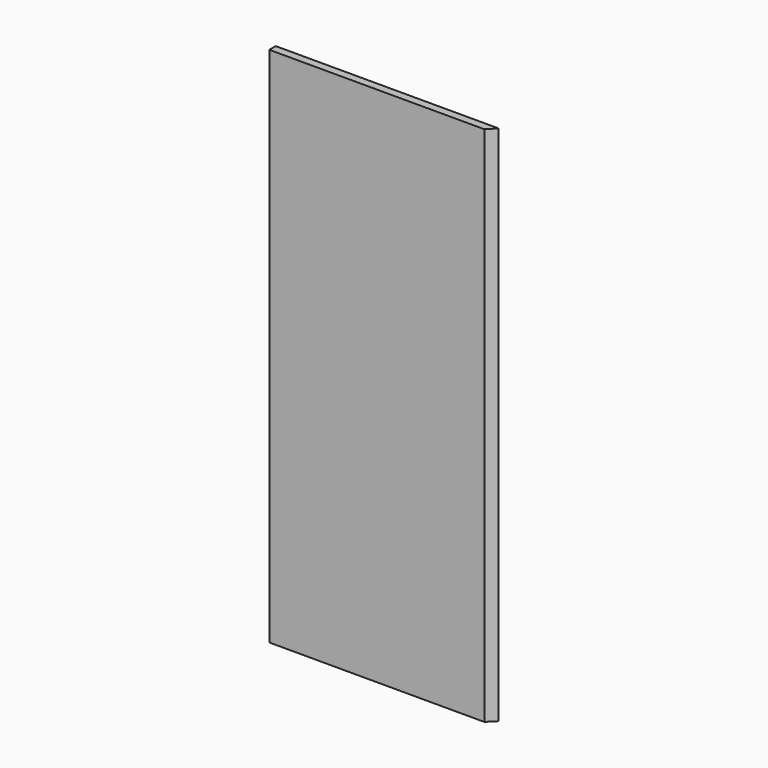
from build123d import *

# Parameters (mm, degrees)
F0_W     = 500
F0_H     = 1170
F1_DEPTH = 18
F2_SIZE  = 17.99999


# Not quite as in the source:
# - a fillet or chamfer is up to 0.001 mm smaller than in the source, because OpenCascade refuses the exact size


with BuildPart() as f1:
    # F0 (on Front) → F1 (new body)
    with BuildSketch(Plane.XZ):
        Rectangle(F0_W, F0_H)
    extrude(amount=F1_DEPTH)

    # F2 (size 18 in the source; OpenCascade refuses exactly that, so slightly less here)
    f2_edges = [f1.edges().sort_by_distance(p)[0] for p in [
        (250, -18, 0),
    ]]
    chamfer(f2_edges, length=F2_SIZE)


solid = f1.part
